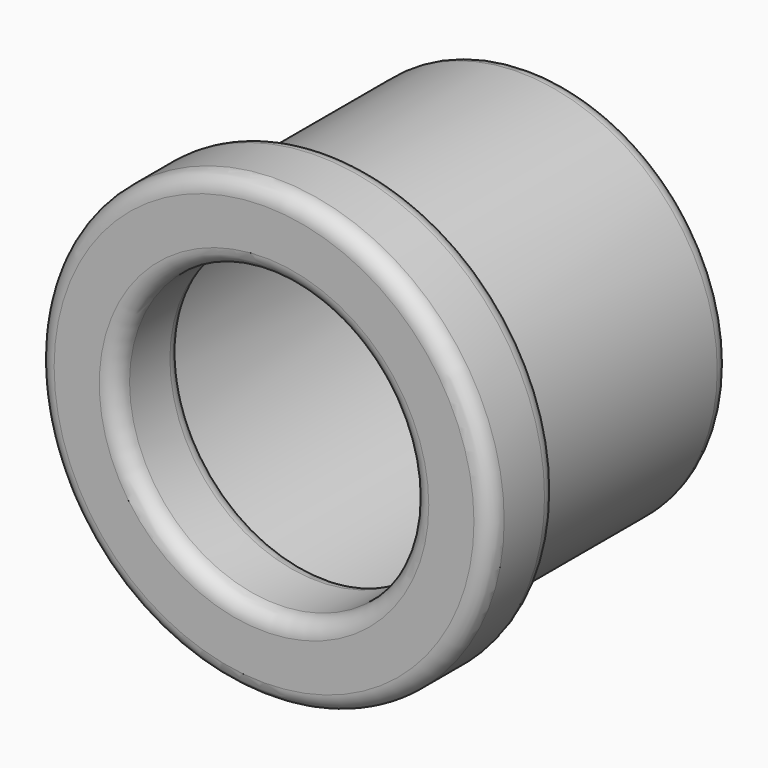
from build123d import *

# Parameters (mm, degrees)
F0_R     = 68.542467708
F0_R_2   = 44.7303954882
F1_DEPTH = 25.4
F2_R     = 5.08
F3_R     = 59.7794080135
F3_R_2   = 55.2190650749
F4_DEPTH = 76.2


# Not quite as in the source:
# - a fillet or chamfer that OpenCascade refuses, or shapes differently, is made with other operations: its cross-section is extruded or revolved along the edge and cut away or added


with BuildPart() as f1:
    # F0 (on Front) → F1 (new body)
    with BuildSketch(Plane.XZ):
        Circle(F0_R)
        Circle(F0_R_2, mode=Mode.SUBTRACT)
    extrude(amount=F1_DEPTH)

    # F2
    f2_edges = [f1.edges().sort_by_distance(p)[0] for p in [
        (-68.542468, -25.4, 0),
        (68.542468, -12.7, 0),
        (-68.542468, 0, 0),
        (-44.730395, -25.4, 0),
        (44.730395, -12.7, 0),
        (-44.730395, 0, 0),
    ]]
    fillet(f2_edges, radius=F2_R)

    # F3 (on Front) → F4 (join)
    with BuildSketch(Plane.XZ):
        Circle(F3_R)
        Circle(F3_R_2, mode=Mode.SUBTRACT)
    extrude(amount=-F4_DEPTH)

    # F5: fillet of radius 5.08 on 3 edges, made by hand

    # F5_s1 → F5_t2 (revolve)
    with BuildSketch(Plane.XY):
        with BuildLine():
            ThreePointArc((64.1609378607, -0.0482468815), (61.028309713, 1.6474777881), (59.7794080135, 4.983506237))
            Line((59.7794080135, 4.983506237), (59.2714080135, 4.983506237))
            Line((59.2714080135, 4.983506237), (59.2714080135, 0))
            Line((59.2714080135, 0), (59.7794080135, -0.508))
            ThreePointArc((59.7794080135, -0.508), (63.462467708, -0.508), (64.0910908454, -0.5514221933))
            Line((64.0910908454, -0.5514221933), (64.1609378607, -0.0482468815))
        make_face()
    revolve(axis=Axis((0, 0, 0), (0, -1, 0)))

    # F5_s3 → F5_t4 (revolve)
    with BuildSketch(Plane.XY):
        with BuildLine():
            ThreePointArc((55.2190650749, 5.08), (53.7311675233, 1.4878975516), (50.1390650749, 0))
            Line((50.1390650749, 0), (55.2190650749, 0))
            Line((55.2190650749, 0), (55.2190650749, 5.08))
        make_face()
    revolve(axis=Axis((0, 0, 0), (0, -1, 0)))

    # F5_s5 → F5_t6 (revolve, cut)
    with BuildSketch(Plane.XY):
        with BuildLine():
            ThreePointArc((59.7794080135, 71.1466489793), (58.4707643923, 74.550069474), (55.2190650749, 76.2))
            Line((55.2190650749, 76.2), (59.7794080135, 76.2))
            Line((59.7794080135, 76.2), (59.7794080135, 71.1466489793))
        make_face()
    revolve(axis=Axis((0, 76.2, 0), (0, -1, 0)), mode=Mode.SUBTRACT)


solid = f1.part
